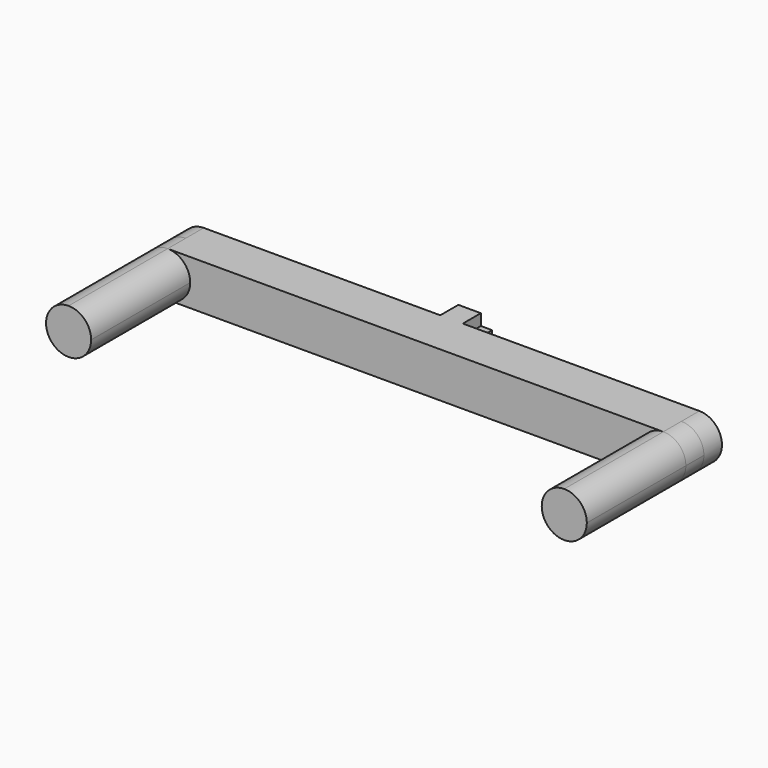
from build123d import *
from build123d import SkipClean  # not in build123d's __all__

# Parameters (mm, degrees)
F1_DEPTH = 82.5
F0_W     = 12.7
F0_H     = 6.35
F2_DEPTH = 12.7
F0_W_2   = 6.35
F0_H_2   = 12.7
F4_DEPTH = 25.4
F5_DEPTH = 12.7


# Not quite as in the source:
# - after a boolean that leaves OpenCascade's solid faulty, fix() repairs it
# - a feature of the source that left no trace in its solid (it failed there, or was rolled back) is left out
# - a feature names something its author has since deleted; it is built from what else it names


with BuildPart() as f1:
    # F0 (on Front) → F1 (new body)
    with BuildSketch(Plane.XZ):
        with BuildLine():
            Line((-139.7, 0), (-139.7, 12.7))
            ThreePointArc((-139.7, 12.7), (-148.6802561211, 8.9802561211), (-152.4, 0))
            Line((-152.4, 0), (-139.7, 0))
        make_face()
        with BuildLine():
            ThreePointArc((-127, 0), (-130.7197438789, 8.9802561211), (-139.7, 12.7))
            Line((-139.7, 12.7), (-139.7, 0))
            Line((-139.7, 0), (-139.7, -12.7))
            ThreePointArc((-139.7, -12.7), (-130.7197438789, -8.9802561211), (-127, 0))
        make_face()
        with BuildLine():
            Line((-139.7, -12.7), (-139.7, 0))
            Line((-139.7, 0), (-152.4, 0))
            ThreePointArc((-152.4, 0), (-148.6802561211, -8.9802561211), (-139.7, -12.7))
        make_face()
        with BuildLine():
            ThreePointArc((-127, 0), (-130.7197438789, 8.9802561211), (-139.7, 12.7))
            Line((-139.7, 12.7), (-139.7, 0))
            Line((-139.7, 0), (-139.7, -12.7))
            ThreePointArc((-139.7, -12.7), (-130.7197438789, -8.9802561211), (-127, 0))
        make_face()
    extrude(amount=F1_DEPTH)



with BuildPart() as f1b:
    # F0 (on Front) → F1, piece 2 (new body)
    with BuildSketch(Plane.XZ):
        with BuildLine():
            Line((139.7, -12.7), (139.7, 12.7))
            ThreePointArc((139.7, 12.7), (127, 0), (139.7, -12.7))
        make_face()
        with BuildLine():
            ThreePointArc((152.4, 0), (148.6802561211, 8.9802561211), (139.7, 12.7))
            Line((139.7, 12.7), (139.7, -12.7))
            ThreePointArc((139.7, -12.7), (148.6802561211, -8.9802561211), (152.4, 0))
        make_face()
        with BuildLine():
            ThreePointArc((152.4, 0), (148.6802561211, 8.9802561211), (139.7, 12.7))
            Line((139.7, 12.7), (139.7, -12.7))
            ThreePointArc((139.7, -12.7), (148.6802561211, -8.9802561211), (152.4, 0))
        make_face()
    extrude(amount=F1_DEPTH)


with BuildPart() as f1_1:
    add(f1.part, clean=False)

    with SkipClean():  # cleaning this boolean's faces spoils the solid; the shape is the same uncleaned
        add(f1b.part)  # F2 merges F1b
    # F0 (on Front) → F2 (join, symmetric)
    with BuildSketch(Plane.XZ):
        with BuildLine():
            Line((139.7, 12.7), (6.35, 12.7))
            Line((6.35, 12.7), (6.35, 6.35))
            Line((6.35, 6.35), (12.7, 6.35))
            Line((12.7, 6.35), (12.7, -6.35))
            Line((12.7, -6.35), (6.35, -6.35))
            Line((6.35, -6.35), (6.35, -12.7))
            Line((6.35, -12.7), (139.7, -12.7))
            ThreePointArc((139.7, -12.7), (127, 0), (139.7, 12.7))
        make_face()
        with BuildLine():
            Line((139.7, -12.7), (139.7, 12.7))
            ThreePointArc((139.7, 12.7), (127, 0), (139.7, -12.7))
        make_face()
        with BuildLine():
            Line((139.7, -12.7), (139.7, 12.7))
            ThreePointArc((139.7, 12.7), (127, 0), (139.7, -12.7))
        make_face()
        with BuildLine():
            ThreePointArc((152.4, 0), (148.6802561211, 8.9802561211), (139.7, 12.7))
            Line((139.7, 12.7), (139.7, -12.7))
            ThreePointArc((139.7, -12.7), (148.6802561211, -8.9802561211), (152.4, 0))
        make_face()
        with BuildLine():
            Line((-139.7, 0), (-139.7, 12.7))
            ThreePointArc((-139.7, 12.7), (-148.6802561211, 8.9802561211), (-152.4, 0))
            Line((-152.4, 0), (-139.7, 0))
        make_face()
        with BuildLine():
            Line((-139.7, -12.7), (-139.7, 0))
            Line((-139.7, 0), (-152.4, 0))
            ThreePointArc((-152.4, 0), (-148.6802561211, -8.9802561211), (-139.7, -12.7))
        make_face()
        with BuildLine():
            ThreePointArc((-127, 0), (-130.7197438789, 8.9802561211), (-139.7, 12.7))
            Line((-139.7, 12.7), (-139.7, 0))
            Line((-139.7, 0), (-139.7, -12.7))
            ThreePointArc((-139.7, -12.7), (-130.7197438789, -8.9802561211), (-127, 0))
        make_face()
        with BuildLine():
            Line((-6.35, 12.7), (-139.7, 12.7))
            ThreePointArc((-139.7, 12.7), (-130.7197438789, 8.9802561211), (-127, 0))
            ThreePointArc((-127, 0), (-130.7197438789, -8.9802561211), (-139.7, -12.7))
            Line((-139.7, -12.7), (-6.35, -12.7))
            Line((-6.35, -12.7), (-6.35, -6.35))
            Line((-6.35, -6.35), (-12.7, -6.35))
            Line((-12.7, -6.35), (-12.7, 6.35))
            Line((-12.7, 6.35), (-6.35, 6.35))
            Line((-6.35, 6.35), (-6.35, 12.7))
        make_face()
        with Locations((0, 9.525)):
            Rectangle(F0_W, F0_H)
    with SkipClean():  # cleaning this boolean's faces spoils the solid; the shape is the same uncleaned
        extrude(amount=F2_DEPTH, both=True)

    # F0 (on Front) → F4 (join)
    with BuildSketch(Plane.XZ):
        with Locations((-9.525, 0)):
            Rectangle(F0_W_2, F0_H_2)
        Rectangle(F0_W, F0_H_2)
        with Locations((0, 9.525)):
            Rectangle(F0_W, F0_H)
        with Locations((9.525, 0)):
            Rectangle(F0_W_2, F0_H_2)
        with Locations((0, -9.525)):
            Rectangle(F0_W, F0_H)
    extrude(amount=-F4_DEPTH)

    add(f1_1.part.fix(), mode=Mode.REPLACE)

    # F0 (on Front) → F5 (join)
    with BuildSketch(Plane.XZ):
        with Locations((9.525, 0)):
            Rectangle(F0_W_2, F0_H_2)
        with Locations((0, -9.525)):
            Rectangle(F0_W, F0_H)
        with Locations((0, 9.525)):
            Rectangle(F0_W, F0_H)
        with Locations((-9.525, 0)):
            Rectangle(F0_W_2, F0_H_2)
        Rectangle(F0_W, F0_H_2)
    extrude(amount=F5_DEPTH)


solid = f1_1.part
